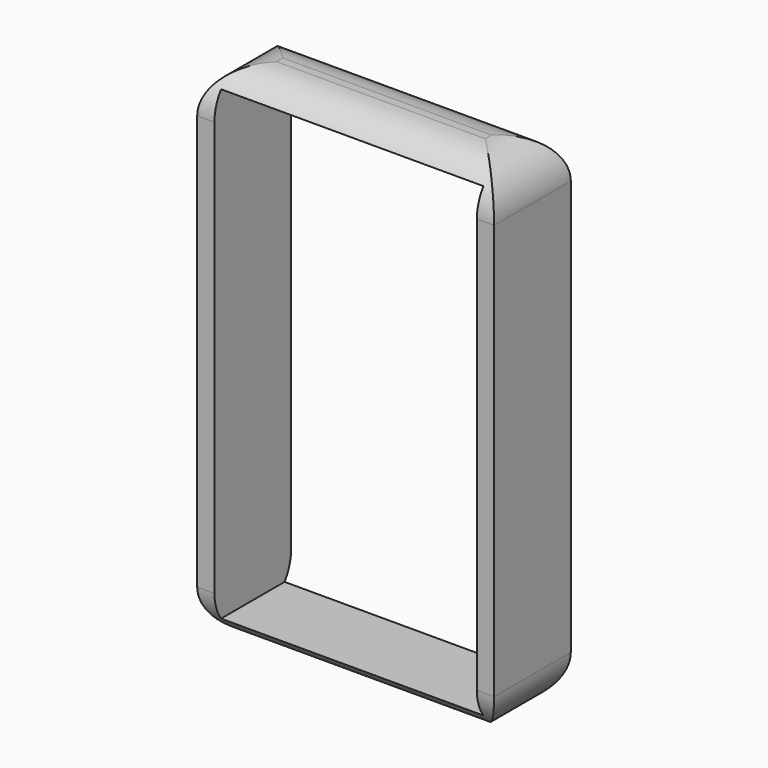
from build123d import *

# Parameters (mm, degrees)
F0_W        = 78.6384046078
F0_H        = 133.1976056099
F0_W_2      = 69.4944038987
F0_H_2      = 123.444005847
F1_DEPTH    = 12.7
F2_T1_DEPTH = 83.6549732601
F2_T3_DEPTH = 136.8933778678


# Not quite as in the source:
# - a fillet or chamfer that OpenCascade refuses, or shapes differently, is made with other operations: its cross-section is extruded or revolved along the edge and cut away or added


with BuildPart() as f1:
    # F0 (on Front) → F1 (new body, symmetric)
    with BuildSketch(Plane.XZ):
        Rectangle(F0_W, F0_H)
        Rectangle(F0_W_2, F0_H_2, mode=Mode.SUBTRACT)
    extrude(amount=F1_DEPTH, both=True)

    # F2: fillet of radius 11.650994652 on 8 edges, made by hand

    # F2_s2 → F2_t1 (cut)
    with BuildSketch(Plane.XZ.offset(-41.82748663)):
        with BuildLine():
            ThreePointArc((39.3192023039, 54.9478081529), (35.9067049779, 63.1863054789), (27.6682076519, 66.5988028049))
            Line((27.6682076519, 66.5988028049), (39.3192023039, 66.5988028049))
            Line((39.3192023039, 66.5988028049), (39.3192023039, 54.9478081529))
        make_face()
        with BuildLine():
            ThreePointArc((-39.3192023039, 54.9478081529), (-35.9067049779, 63.1863054789), (-27.6682076519, 66.5988028049))
            Line((-27.6682076519, 66.5988028049), (-39.3192023039, 66.5988028049))
            Line((-39.3192023039, 66.5988028049), (-39.3192023039, 54.9478081529))
        make_face()
        with BuildLine():
            ThreePointArc((39.3192023039, -54.9478081529), (35.9067049779, -63.1863054789), (27.6682076519, -66.5988028049))
            Line((27.6682076519, -66.5988028049), (39.3192023039, -66.5988028049))
            Line((39.3192023039, -66.5988028049), (39.3192023039, -54.9478081529))
        make_face()
        with BuildLine():
            ThreePointArc((-27.6682076519, -66.5988028049), (-35.9067049779, -63.1863054789), (-39.3192023039, -54.9478081529))
            Line((-39.3192023039, -54.9478081529), (-39.3192023039, -66.5988028049))
            Line((-39.3192023039, -66.5988028049), (-27.6682076519, -66.5988028049))
        make_face()
    extrude(amount=F2_T1_DEPTH, mode=Mode.SUBTRACT)

    # F2_s4 → F2_t3 (cut)
    with BuildSketch(Plane.YZ.offset(-68.4466889339)):
        with BuildLine():
            ThreePointArc((1.049005348, 66.5988028049), (9.287502674, 63.1863054789), (12.7, 54.9478081529))
            Line((12.7, 54.9478081529), (12.7, 66.5988028049))
            Line((12.7, 66.5988028049), (1.049005348, 66.5988028049))
        make_face()
        with BuildLine():
            ThreePointArc((-12.7, 54.9478081529), (-9.287502674, 63.1863054789), (-1.049005348, 66.5988028049))
            Line((-1.049005348, 66.5988028049), (-12.7, 66.5988028049))
            Line((-12.7, 66.5988028049), (-12.7, 54.9478081529))
        make_face()
        with BuildLine():
            ThreePointArc((1.049005348, -66.5988028049), (9.287502674, -63.1863054789), (12.7, -54.9478081529))
            Line((12.7, -54.9478081529), (12.7, -66.5988028049))
            Line((12.7, -66.5988028049), (1.049005348, -66.5988028049))
        make_face()
        with BuildLine():
            ThreePointArc((-1.049005348, -66.5988028049), (-9.287502674, -63.1863054789), (-12.7, -54.9478081529))
            Line((-12.7, -54.9478081529), (-12.7, -66.5988028049))
            Line((-12.7, -66.5988028049), (-1.049005348, -66.5988028049))
        make_face()
    extrude(amount=F2_T3_DEPTH, mode=Mode.SUBTRACT)


solid = f1.part
